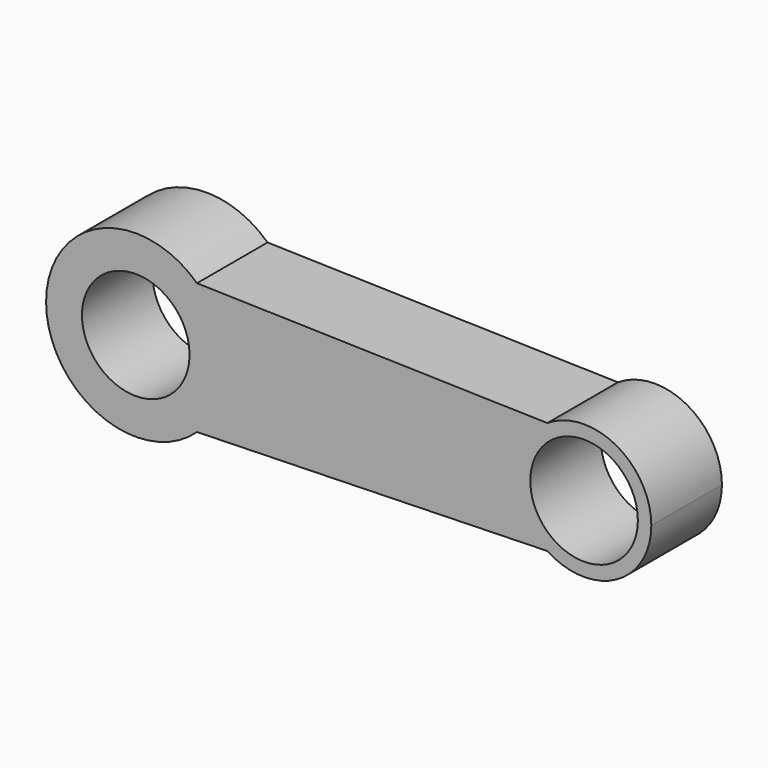
from build123d import *

# Parameters (mm, degrees)
F0_R     = 15.24
F1_DEPTH = 25


# Not quite as in the source:
# - a feature names something its author has since deleted; it is built from what else it names


with BuildPart() as f1:
    # F0 (on Front) → F1 (new body)
    with BuildSketch(Plane.XZ):
        with BuildLine():
            ThreePointArc((17.3446724068, 18.5559246361), (23.2992991218, 10.1144777637), (25.4, 0))
            ThreePointArc((25.4, 0), (23.2992991218, -10.1144777637), (17.3446724068, -18.5559246361))
            Line((17.3446724068, -18.5559246361), (116.5943626679, -15.9569800311))
            ThreePointArc((116.5943626679, -15.9569800311), (107.95, 0), (116.5943626679, 15.9569800311))
            Line((116.5943626679, 15.9569800311), (17.3446724068, 18.5559246361))
        make_face()
        with BuildLine():
            ThreePointArc((17.3446724068, -18.5559246361), (23.2992991218, -10.1144777637), (25.4, 0))
            ThreePointArc((25.4, 0), (23.2992991218, 10.1144777637), (17.3446724068, 18.5559246361))
            ThreePointArc((17.3446724068, 18.5559246361), (-25.4, 0), (17.3446724068, -18.5559246361))
        make_face()
        Circle(F0_R, mode=Mode.SUBTRACT)
        with BuildLine():
            ThreePointArc((146.05, 0), (136.0740043207, 16.7500730025), (116.5943626679, 15.9569800311))
            ThreePointArc((116.5943626679, 15.9569800311), (107.95, 0), (116.5943626679, -15.9569800311))
            ThreePointArc((116.5943626679, -15.9569800311), (136.0740043207, -16.7500730025), (146.05, 0))
        make_face()
        with Locations((127, 0)):
            Circle(F0_R, mode=Mode.SUBTRACT)
    extrude(amount=F1_DEPTH)


solid = f1.part
